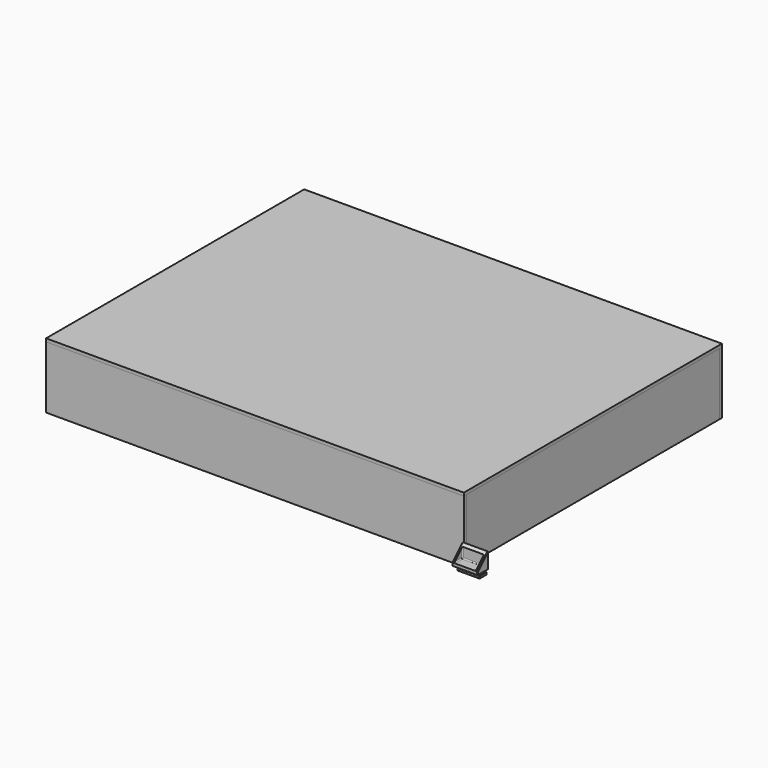
from build123d import *

# Parameters (mm, degrees)
F0_W      = 23
F0_H      = 8.5
F1_DEPTH  = 3
F2_W      = 4.5
F2_H      = 5
F3_DEPTH  = 2.85
F4_W      = 26
F4_H      = 13
F5_DEPTH  = 3
F7_DEPTH  = 26
F8_SIZE   = 0.5
F9_R      = 0.25
F10_SIZE  = 0.5
F12_DEPTH = 63.5
F11_W     = 3.175
F11_H     = 322.65
F13_DEPTH = 63.5
F14_W     = 426
F14_H     = 329
F15_DEPTH = 3.175
F17_START = -2
F17_DEPTH = 22
F18_SIZE  = 0.5
F19_R     = 1


# Not quite as in the source:
# - a length typed as a fraction of an inch, garbled in the dataset ("3 / 203.2 mm" for 3/8 in), is restored


with BuildPart() as f1:
    # F0 (on Top) → F1 (new body)
    with BuildSketch(Plane.XY):
        with Locations((11.5, 4.25)):
            Rectangle(F0_W, F0_H)
    extrude(amount=F1_DEPTH)

    # F2 (on face) → F3 (join)
    with BuildSketch(Plane.XY.offset(3)):
        with Locations((6.825, 6)):
            Rectangle(F2_W, F2_H)
        with Locations((16.175, 6)):
            Rectangle(F2_W, F2_H)
    extrude(amount=F3_DEPTH)

    # F4 (on face) → F5 (join)
    with BuildSketch(Plane.XY.offset(5.85)):
        with Locations((11.5, 2)):
            Rectangle(F4_W, F4_H)
    extrude(amount=F5_DEPTH)

    # F6 (on face) → F7 (join, through all)
    with BuildSketch(Plane.YZ.offset(24.5)):
        Polygon((-4.5, 8.85), (8.5, 8.85), (8.5, 21.85), align=None)
    extrude(amount=-F7_DEPTH)

    # F8
    f8_edges = [f1.edges().sort_by_distance(p)[0] for p in [
        (4.575, 3.5, 4.425),
        (9.075, 3.5, 4.425),
        (13.925, 3.5, 4.425),
        (18.425, 3.5, 4.425),
    ]]
    chamfer(f8_edges, length=F8_SIZE)

    # F9
    f9_edges = [f1.edges().sort_by_distance(p)[0] for p in [
        (4.575, 6.25, 5.85),
        (4.825, 3.75, 5.85),
        (6.825, 3.5, 5.85),
        (8.825, 3.75, 5.85),
        (9.075, 6.25, 5.85),
        (13.925, 6.25, 5.85),
        (14.175, 3.75, 5.85),
        (16.175, 3.5, 5.85),
        (18.175, 3.75, 5.85),
        (18.425, 6.25, 5.85),
        (18.425, 6.25, 3),
        (18.175, 3.75, 3),
        (16.175, 3.5, 3),
        (14.175, 3.75, 3),
        (13.925, 6.25, 3),
        (6.825, 3.5, 3),
        (4.825, 3.75, 3),
        (4.575, 6.25, 3),
        (8.825, 3.75, 3),
        (9.075, 6.25, 3),
    ]]
    fillet(f9_edges, radius=F9_R)

    # F10
    f10_edges = [f1.edges().sort_by_distance(p)[0] for p in [
        (0, 4.25, 3),
        (0, 0, 1.5),
        (0, 4.25, 0),
        (11.5, 0, 3),
        (11.5, 0, 0),
        (23, 4.25, 3),
        (23, 0, 1.5),
        (23, 4.25, 0),
    ]]
    chamfer(f10_edges, length=F10_SIZE)

    # F16 (on face) → F17 (cut)
    with BuildSketch(Plane.YZ.offset(24.5).offset(F17_START)):
        Polygon((6, 19.35), (-4.5, 8.85), (6, 8.85), align=None)
    extrude(amount=-F17_DEPTH, mode=Mode.SUBTRACT)

    # F18
    f18_edges = [f1.edges().sort_by_distance(p)[0] for p in [
        (24.5, 2, 15.35),
        (24.5, -4.5, 7.35),
        (-1.5, -4.5, 7.35),
        (-1.5, 2, 15.35),
    ]]
    chamfer(f18_edges, length=F18_SIZE)

    # F19
    f19_edges = [f1.edges().sort_by_distance(p)[0] for p in [
        (11.5, 6, 8.85),
        (0.5, 6, 14.1),
        (0.5, 0.75, 8.85),
        (22.5, 6, 14.1),
        (22.5, 0.75, 8.85),
    ]]
    fillet(f19_edges, radius=F19_R)


with BuildPart() as f12:
    # F11 (on Top) → F12 (new body)
    with BuildSketch(Plane.XY):
        Polygon((-426, 8.5), (0, 8.5), (0, 11.675), (-3.175, 11.675), (-422.825, 11.675), (-426, 11.675), align=None)
    extrude(amount=F12_DEPTH)


with BuildPart() as f12b:
    # F11 (on Top) → F12, piece 2 (new body)
    with BuildSketch(Plane.XY):
        Polygon((-3.175, 334.325), (0, 334.325), (0, 337.5), (-426, 337.5), (-426, 334.325), (-422.825, 334.325), align=None)
    extrude(amount=F12_DEPTH)


with BuildPart() as f13:
    # F11 (on Top) → F13 (new body, through all)
    with BuildSketch(Plane.XY):
        with Locations((-1.5875, 173)):
            Rectangle(F11_W, F11_H)
    extrude(amount=F13_DEPTH)


with BuildPart() as f13b:
    # F11 (on Top) → F13, piece 2 (new body, through all)
    with BuildSketch(Plane.XY):
        with Locations((-424.4125, 173)):
            Rectangle(F11_W, F11_H)
    extrude(amount=F13_DEPTH)


with BuildPart() as f15:
    # F14 (on face) → F15 (new body)
    with BuildSketch(Plane.XY.offset(63.5)):
        with Locations((-213, 173)):
            Rectangle(F14_W, F14_H)
    extrude(amount=F15_DEPTH)


solid = Compound([f1.part, f12.part, f12b.part, f13.part, f13b.part, f15.part])
